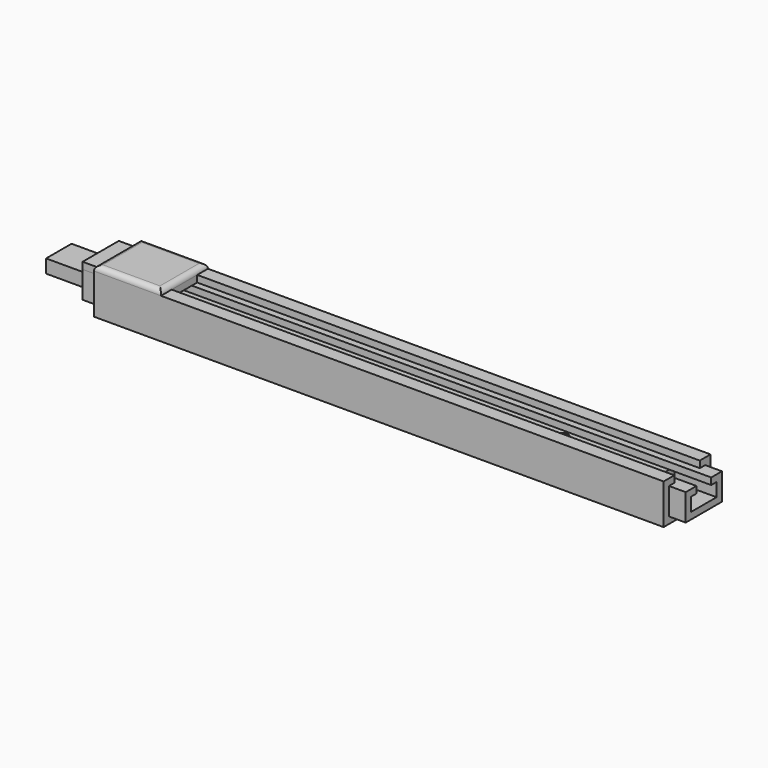
from build123d import *

# Parameters (mm, degrees)
F0_W      = 360
F0_H      = 19
F0_R      = 4
F1_DEPTH  = 8
F4_DEPTH  = 360
F7_DEPTH  = 340
F8_W      = 50
F8_H      = 11
F9_DEPTH  = 4
F10_W     = 40
F10_H     = 8
F10_H_2   = 19
F11_DEPTH = 3
F12_R     = 2.99999
F13_R     = 4
F14_DEPTH = 4


# Not quite as in the source:
# - a fillet or chamfer is up to 0.001 mm smaller than in the source, because OpenCascade refuses the exact size


with BuildPart() as f1:
    # F0 (on Top) → F1 (new body)
    with BuildSketch(Plane.XY):
        with Locations((180, 9.5)):
            Rectangle(F0_W, F0_H)
        with Locations((300, 9.5)):
            Circle(F0_R, mode=Mode.SUBTRACT)
    extrude(amount=F1_DEPTH)


with BuildPart() as f4:
    # F3 (on offset) → F4 (new body)
    with BuildSketch(Plane(origin=(25, 0, 0), x_dir=(0, -1, 0), z_dir=(-1, 0, 0))):
        Polygon((0, 0), (-19, 0), (-19, 8), (-15, 8), (-15, 12), (-23, 12), (-23, -4), (4, -4), (4, 12), (-4, 12), (-4, 8), (0, 8), align=None)
    extrude(amount=-F4_DEPTH)

    # F13 (on face) → F14 (cut)
    with BuildSketch(Plane.XY):
        with Locations((367, 9.5)):
            Circle(F13_R)
    extrude(amount=-F14_DEPTH, mode=Mode.SUBTRACT)


with BuildPart() as f7:
    # F6 (on offset) → F7 (new body)
    with BuildSketch(Plane(origin=(35, 0, 0), x_dir=(0, -1, 0), z_dir=(-1, 0, 0))):
        Polygon((-27, 16), (-27, -8), (8, -8), (8, 16), (0, 16), (0, 12), (4, 12), (4, -4), (-23, -4), (-23, 12), (-19, 12), (-19, 16), align=None)
    extrude(amount=-F7_DEPTH)


with BuildPart() as f9:
    # F8 (on face) → F9 (new body)
    with BuildSketch(Plane.XY.offset(12)):
        Polygon((35, 23), (25, 23), (25, 15), (75, 15), (75, 19), (35, 19), align=None)
        with Locations((50, 9.5)):
            Rectangle(F8_W, F8_H)
        Polygon((75, 4), (25, 4), (25, -4), (35, -4), (35, 0), (75, 0), align=None)
    extrude(amount=F9_DEPTH)


with BuildPart() as f11:
    # F10 (on face) → F11 (new body)
    with BuildSketch(Plane.XY.offset(16)):
        with Locations((55, 23)):
            Rectangle(F10_W, F10_H)
        with Locations((55, 9.5)):
            Rectangle(F10_W, F10_H_2)
        with Locations((55, -4)):
            Rectangle(F10_W, F10_H)
    extrude(amount=F11_DEPTH)

    # F12 (radius 3 in the source; OpenCascade refuses exactly that, so slightly less here)
    f12_edges = [f11.edges().sort_by_distance(p)[0] for p in [
        (55, -8, 19),
        (35, 9.5, 19),
        (55, 27, 19),
        (75, 9.5, 19),
    ]]
    fillet(f12_edges, radius=F12_R)


solid = Compound([f1.part, f4.part, f7.part, f9.part, f11.part])
